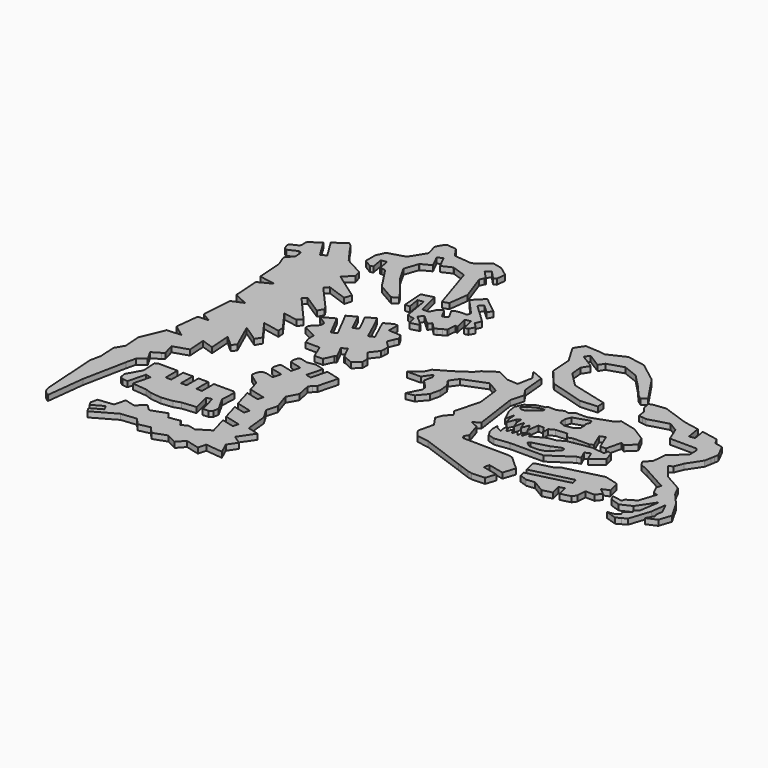
from build123d import *

# Parameters (mm, degrees)
F1_DEPTH = 3


# Not quite as in the source:
# - ends of sketch curves that miss each other by under 0.0002 mm in the source are joined


with BuildPart() as f1:
    # F0 (on Top) → F1 (new body)
    with BuildSketch(Plane.XY):
        Polygon((-104.437403, 46.564107), (-93.530615, 42.688137), (-92.321369, 46.634252), (-107.328489, 57.252365), (-102.324044, 61.359671), (-103.458085, 65.467584), (-113.663104, 70.984544), (-120.264377, 80.128426), (-120.756849, 80.974135), (-121.389462, 81.894522), (-122.514574, 83.041283), (-123.728328, 84.002663), (-130.063193, 79.125245), (-123.876212, 69.030337), (-126.463505, 67.191431), (-132.650487, 77.286339), (-137.732799, 73.674062), (-138.217282, 73.320664), (-138.526723, 72.785836), (-138.607686, 72.16178), (-138.468659, 70.035609), (-138.546917, 69.419841), (-138.847826, 68.889483), (-139.320957, 68.533506), (-142.435409, 67.101481), (-143.009225, 66.616569), (-143.281047, 65.887651), (-143.177988, 65.110044), (-142.393729, 63.132037), (-141.943435, 62.514076), (-141.266561, 62.221382), (-140.544494, 62.332335), (-136.10605, 64.373171), (-135.450674, 64.491083), (-134.818024, 64.272478), (-134.348725, 63.766009), (-134.147103, 63.084244), (-133.962555, 60.261903), (-134.064128, 59.580358), (-134.435555, 59.017782), (-136.792349, 56.777013), (-137.140032, 56.273256), (-137.268685, 55.661094), (-137.156299, 55.045254), (-135.022563, 49.646019), (-134.109418, 35.681092), (-125.140274, 34.118445), (-132.367969, 30.42543), (-131.412679, 15.815968), (-123.662433, 12.327511), (-129.911486, 9.725252), (-131.078484, -6.919091), (-125.924777, -10.012076), (-131.710451, -10.450802), (-133.125015, -23.174873), (-126.622962, -28.006874), (-134.303943, -28.589321), (-139.624962, -41.24429), (-138.992784, -50.912317), (-141.863543, -55.764821), (-141.271361, -64.821195), (-142.540436, -70.997637), (-140.515428, -101.966537), (-140.228003, -103.498246), (-139.58695, -104.900216), (-138.634739, -106.079438), (-137.434522, -106.957791), (-136.483255, -107.475311), (-134.012522, -86.428392), (-129.312015, -62.860274), (-128.020019, -57.445451), (-123.992793, -54.409686), (-127.09608, -48.956719), (-122.790594, -46.396882), (-121.548537, -45.29548), (-123.317555, -38.886306), (-115.18349, -36.282735), (-115.824054, -26.486441), (-109.192589, -28.71396), (-109.962426, -16.940676), (-104.125971, -22.186389), (-102.289088, -19.816338), (-108.825287, -5.250342), (-99.761113, -11.388933), (-97.77603, -7.98978), (-105.76927, 2.944957), (-96.452884, 1.068715), (-96.675299, 4.470164), (-104.586688, 15.321374), (-96.764237, 13.866803), (-94.584782, 16.079816), (-107.600103, 30.944294), (-105.732261, 32.840884), (-95.236183, 26.041835), (-93.454355, 29.231747), (-94.801805, 31.363182), (-106.496474, 44.528166), align=None)
    extrude(amount=F1_DEPTH)


with BuildPart() as f1b:
    # F0 (on Top) → F1, piece 2 (new body)
    with BuildSketch(Plane.XY):
        Polygon((-89.056032, 108.81387), (-89.684225, 108.642768), (-90.249705, 108.36248), (-90.766267, 107.966165), (-91.049446, 107.379957), (-92.740363, 104.245862), (-92.761765, 103.761682), (-92.617803, 103.298892), (-91.094478, 97.874397), (-96.342567, 89.382437), (-105.576906, 86.652048), (-107.737054, 81.985061), (-107.81263, 75.445893), (-103.524276, 72.84311), (-101.918124, 73.309127), (-103.032279, 79.807423), (-99.976868, 80.331274), (-98.921946, 74.178449), (-98.329958, 74.350211), (-95.800781, 73.792723), (-87.539001, 61.142449), (-83.059492, 58.556348), (-81.325187, 57.555105), (-78.121592, 55.705613), (-75.268916, 57.618377), (-77.57377, 61.251598), (-85.793508, 71.451888), (-90.559396, 79.785333), (-88.012588, 87.248984), (-87.488279, 87.697366), (-82.649191, 90.248926), (-85.944045, 96.896256), (-83.166522, 98.272979), (-79.871667, 91.625648), (-74.910829, 93.931576), (-74.236509, 94.077314), (-66.570524, 91.461465), (-58.372939, 65.993132), (-55.12332, 67.105068), (-53.747377, 77.891799), (-58.811761, 92.126912), (-57.723892, 94.477245), (-57.228728, 94.844348), (-57.275961, 94.894994), (-61.486422, 99.409668), (-59.219354, 101.523988), (-54.722596, 96.702332), (-53.37914, 97.698335), (-52.853684, 102.687158), (-54.477515, 103.893374), (-58.148833, 106.620508), (-63.146548, 107.678315), (-70.890179, 101.998314), (-80.826131, 102.964066), (-83.931775, 107.573558), (-84.212894, 107.968363), (-84.611172, 108.244523), (-88.418044, 108.684252), align=None)
    extrude(amount=F1_DEPTH)


with BuildPart() as f1c:
    # F0 (on Top) → F1, piece 3 (new body)
    with BuildSketch(Plane.XY):
        Polygon((-42.159712, 46.354486), (-40.319081, 47.369456), (-40.319496, 48.757673), (-40.035886, 52.328733), (-38.747849, 52.100388), (-38.657511, 52.126978), (-40.238607, 59.075176), (-37.215885, 59.763052), (-35.677786, 53.003806), (-33.794305, 53.558068), (-32.126363, 56.540318), (-34.89486, 59.272544), (-33.499978, 62.572179), (-38.761047, 67.63558), (-44.111875, 72.599139), (-42.003621, 74.871866), (-37.16445, 70.38293), (-35.646276, 72.995292), (-44.68013, 80.268067), (-50.226429, 74.695501), (-41.7868, 65.424247), (-42.380248, 63.371775), (-46.1018, 63.329178), (-48.125943, 62.914547), (-49.899462, 61.936585), (-47.046077, 56.762013), (-49.760707, 55.2651), (-52.614093, 60.439672), (-55.149767, 59.041439), (-56.932791, 55.347147), (-60.497214, 55.106867), (-63.550508, 67.348278), (-69.896804, 65.765349), (-69.05246, 53.912434), (-66.451193, 54.097766), (-67.567519, 60.669727), (-64.511289, 61.18887), (-62.162859, 47.517114), (-59.954925, 46.624454), (-59.968276, 46.648665), (-58.196369, 46.423521), (-57.009088, 42.030694), (-52.478271, 43.255272), (-52.267646, 43.553602), (-58.01691, 48.767286), (-55.934437, 51.063668), (-50.466297, 46.104917), (-49.090656, 48.053332), (-45.641155, 44.434734), (-44.429485, 45.102878), align=None)
    extrude(amount=F1_DEPTH)


with BuildPart() as f1d:
    # F0 (on Top) → F1, piece 4 (new body)
    with BuildSketch(Plane.XY):
        Polygon((-50.048866, 4.568951), (-53.825765, 9.290101), (-50.257894, 13.877362), (-50.048866, 16.092855), (-50.048866, 18.597474), (-53.825765, 22.374398), (-52.443705, 25.522427), (-51.397753, 27.904872), (-52.881541, 30.602621), (-59.49114, 31.007296), (-59.49114, 37.044992), (-61.447204, 37.044992), (-65.93857, 34.588814), (-60.398711, 22.505428), (-63.216676, 21.213468), (-68.665206, 33.097653), (-70.587792, 36.613251), (-75.208392, 34.086347), (-70.405513, 24.338759), (-73.186282, 22.968586), (-77.930728, 32.597564), (-82.763, 29.954908), (-81.268778, 27.222657), (-75.0956, 15.246371), (-77.851086, 13.826037), (-83.989445, 25.734784), (-90.380846, 22.239498), (-85.389947, 18.867223), (-85.389947, 16.574149), (-89.166846, 12.662325), (-89.166846, 10.639), (-81.747923, 7.131876), (-81.747923, 3.354952), (-80.53391, -0.017323), (-78.334601, -0.017323), (-76.277469, -0.017323), (-72.845212, -0.017323), (-69.74275, -7.436196), (-65.156501, -7.436196), (-62.863376, -2.310397), (-61.921049, -1.758048), (-65.426718, 5.301226), (-62.650225, 6.680051), (-59.240248, -0.186524), (-58.951577, -0.017323), (-53.825765, -2.310397), (-50.048866, 0.926927), align=None)
    extrude(amount=F1_DEPTH)


with BuildPart() as f1e:
    # F0 (on Top) → F1, piece 5 (new body)
    with BuildSketch(Plane.XY):
        Polygon((-75.430288, -23.271141), (-76.058576, -23.64166), (-76.264869, -23.909784), (-77.0207, -26.614304), (-77.013935, -27.343677), (-76.643403, -27.971962), (-76.008398, -28.330798), (-70.103598, -29.854618), (-71.240521, -34.260194), (-75.780919, -33.088478), (-76.878802, -33.0267), (-77.916726, -33.389771), (-78.736739, -34.122396), (-79.213925, -35.113052), (-79.74799, -37.182556), (-79.777736, -37.739591), (-79.588947, -38.264513), (-79.211233, -38.675058), (-73.457518, -42.851059), (-71.659574, -49.055771), (-62.769283, -51.35004), (-63.543907, -54.351707), (-70.656943, -52.516085), (-67.731057, -62.613493), (-59.56419, -64.721072), (-60.338813, -67.722734), (-66.728377, -66.073814), (-64.030647, -75.384005), (-55.411149, -77.608391), (-56.185772, -80.610053), (-63.027965, -78.844325), (-60.176841, -88.80404), (-67.161825, -93.110121), (-71.126836, -92.086892), (-74.615758, -93.770966), (-76.854063, -90.608898), (-82.986358, -91.610812), (-85.224663, -88.448743), (-93.74448, -91.418951), (-97.304474, -87.915814), (-99.0472, -89.68684), (-101.372527, -92.049925), (-107.149621, -90.559062), (-108.737669, -96.712747), (-116.966109, -97.643601), (-117.932495, -101.388347), (-116.718659, -103.538261), (-110.605866, -100.087016), (-109.081749, -102.786491), (-115.194543, -106.237737), (-113.740062, -108.81387), (-101.173814, -101.719032), (-92.657288, -100.862523), (-89.431274, -104.749365), (-82.965051, -103.363745), (-79.739037, -107.250587), (-72.491108, -104.657004), (-66.664429, -107.570357), (-63.047577, -103.569816), (-55.558085, -105.502588), (-54.421162, -101.097011), (-45.048666, -102.106025), (-47.848312, -95.838753), (-44.522848, -90.964192), (-49.278536, -87.719779), (-43.577011, -79.362376), (-49.68623, -77.785803), (-50.953558, -65.809785), (-54.385668, -59.990156), (-52.793977, -53.822356), (-55.707329, -45.082272), (-52.573661, -39.312395), (-54.115483, -31.663113), (-52.822456, -29.959439), (-51.223581, -28.618216), (-48.381276, -17.604286), (-51.163921, -16.886184), (-56.100521, -15.612223), (-58.356868, -24.355565), (-61.358527, -23.580943), (-59.102181, -14.837601), (-64.241319, -13.511372), (-66.810155, -13.998182), (-68.440858, -14.30721), (-72.142864, -13.351854), (-72.872212, -13.3586), (-73.500502, -13.729123), (-73.859368, -14.364144), (-74.462625, -16.701766), (-74.455861, -17.431139), (-74.085327, -18.05942), (-73.450323, -18.418259), (-67.545523, -19.942079), (-68.796138, -24.78821), (-74.700938, -23.264391), align=None)
    extrude(amount=F1_DEPTH)


with BuildPart() as f1f:
    # F0 (on Top) → F1, piece 6 (new body)
    with BuildSketch(Plane.XY):
        Polygon((-95.511904, -55.049836), (-95.512207, -63.250328), (-98.62354, -63.249836), (-98.622245, -55.049836), (-103.974963, -55.04899), (-103.976256, -63.233232), (-107.088527, -63.232729), (-107.087234, -55.048474), (-117.855523, -55.046772), (-119.091081, -55.832964), (-119.023882, -57.066132), (-118.908188, -59.189267), (-118.649276, -63.940604), (-122.921193, -71.627557), (-122.479558, -74.714973), (-120.877028, -75.844105), (-117.779126, -76.120585), (-115.302533, -66.371024), (-112.297975, -67.134254), (-114.651594, -76.39971), (-106.771164, -77.10302), (-103.128968, -78.336641), (-97.067074, -78.982632), (-91.00518, -78.336641), (-87.362985, -77.10302), (-79.482554, -76.39971), (-81.836173, -67.134254), (-78.831616, -66.371024), (-76.355023, -76.120585), (-73.257121, -75.844105), (-71.654591, -74.714973), (-71.212956, -71.627557), (-75.484872, -63.940604), (-75.043068, -55.832964), (-76.278625, -55.046772), (-87.046915, -55.048474), (-87.045621, -63.232729), (-90.157892, -63.233232), (-90.159186, -55.04899), align=None)
    extrude(amount=F1_DEPTH)


with BuildPart() as f1g:
    # F0 (on Top) → F1, piece 7 (new body)
    with BuildSketch(Plane.XY):
        Polygon((8.495949, -34.135969), (11.346512, -37.863053), (18.082474, -38.978129), (41.668499, -47.500932), (43.705116, -48.236862), (48.891428, -50.110934), (51.389669, -50.656791), (58.502406, -50.387424), (60.309291, -44.858784), (51.909904, -42.937152), (52.601264, -39.915215), (61.27627, -41.8999), (63.45597, -35.230399), (55.734619, -28.208075), (53.264095, -27.631666), (27.938087, -27.412399), (27.104545, -25.680222), (28.415999, -23.513753), (25.785276, -15.325359), (21.698488, -13.430989), (25.160498, -11.085757), (21.745718, 12.957322), (23.712684, 20.155122), (20.837889, 24.398867), (19.659859, 36.960822), (13.016846, 39.792383), (16.421207, 34.766897), (14.872141, 26.711679), (8.996459, 26.967452), (1.71219, 30.505123), (-4.876789, 26.041621), (-7.027485, 23.444219), (-14.398211, 18.451147), (-22.258862, 13.940791), (-23.620617, 10.900292), (-29.344982, 5.881985), (-21.93824, 6.011688), (-18.717606, 10.637306), (-17.582814, 8.962138), (-18.631145, 4.015904), (-14.106414, -0.739377), (-13.865017, -3.019809), (-17.478357, -10.192355), (-13.032845, -9.298961), (-8.7675, -4.291452), (-7.499394, 1.292387), (-7.94972, 6.52685), (-10.521909, 10.323891), (-7.448974, 14.686517), (5.159795, 19.643562), (11.435362, 15.911362), (12.948402, 3.57641), (9.345901, -10.105917), (11.388524, -13.121218), (8.256665, -16.248632), (6.818535, -20.090334), (10.510365, -25.540178), align=None)
    extrude(amount=F1_DEPTH)


with BuildPart() as f1h:
    # F0 (on Top) → F1, piece 8 (new body)
    with BuildSketch(Plane.XY):
        Polygon((46.31628, 74.243386), (36.435113, 76.041081), (32.979415, 74.41313), (31.25546, 73.60099), (26.861843, 71.531194), (23.451776, 72.049742), (15.694626, 72.513066), (12.388123, 67.488849), (18.404778, 57.332014), (19.164542, 45.733344), (26.766633, 36.64906), (45.655597, 31.14136), (54.887635, 31.772631), (54.588393, 35.997475), (34.948236, 41.071774), (27.038098, 48.984554), (26.513995, 55.362823), (28.986028, 59.29483), (21.286694, 64.135364), (22.936641, 66.759792), (30.635984, 61.919269), (32.539838, 64.947517), (41.341244, 67.724972), (49.551788, 64.506242), (56.573036, 57.271918), (62.09137, 50.832995), (64.609843, 48.910836), (67.255221, 50.994557), (57.279075, 65.876312), align=None)
    extrude(amount=F1_DEPTH)


with BuildPart() as f1i:
    # F0 (on Top) → F1, piece 9 (new body)
    with BuildSketch(Plane.XY):
        Polygon((41.50084, -4.359526), (43.008741, -0.46998), (43.68228, -1.009414), (45.119556, -4.359526), (46.019556, 1.951114), (49.058002, 1.951114), (51.395266, -1.554777), (51.395266, 1.951114), (54.199987, 3.431378), (60.354797, 3.976741), (62.458336, 1.016213), (65.496782, 1.951114), (68.825445, 1.951114), (71.163095, 1.951114), (74.300488, 1.951114), (75.867294, 2.789517), (72.620786, 10.525798), (75.462236, 11.718197), (78.960044, 3.383076), (82.013472, 3.431378), (84.039104, 11.767645), (86.064737, 10.59903), (90.661362, 15.039822), (87.934551, 20.415561), (80.377386, 25.167957), (71.339949, 27.349454), (69.080591, 25.167957), (67.033284, 24.443741), (61.209136, 22.383503), (57.627983, 21.116703), (51.473178, 21.116703), (48.980089, 19.013187), (46.487006, 19.714374), (43.02313, 18.078286), (38.462388, 18.078286), (37.917025, 17.221274), (36.313726, 16.840829), (35.521631, 16.652874), (33.320403, 16.130548), (28.9575, 13.17002), (27.087686, 9.118721), (27.358255, 7.224767), (27.710961, 4.755863), (30.784317, -1.851861), (32.072677, 3.04184), (32.38549, -1.009414), (33.398304, -4.359526), (35.190217, 0.427862), (36.904212, 1.951114), (36.904212, -1.554777), (38.384481, -5.13858), (39.708932, 0.315026), align=None)
        Polygon((29.249174, 10.309388), (31.293509, 12.503303), (35.830915, 14.796977), (36.632082, 14.930491), (38.822621, 15.295543), (38.822621, 14.198562), (38.024831, 13.301053), (32.340599, 9.15972), (30.482975, 9.15972), align=None, mode=Mode.SUBTRACT)
        Polygon((51.33145, 13.950375), (52.488246, 16.782518), (61.209136, 19.603975), (61.981914, 17.739882), (61.024573, 15.545967), (61.622908, 14.548699), (61.622908, 11.51713), (58.910436, 9.56259), (54.522605, 8.764748), (51.810126, 10.001345), (51.33145, 11.51713), align=None, mode=Mode.SUBTRACT)
    extrude(amount=F1_DEPTH)


with BuildPart() as f1j:
    # F0 (on Top) → F1, piece 10 (new body)
    with BuildSketch(Plane.XY):
        Polygon((51.059302, -18.357568), (59.964344, -18.357568), (65.195759, -18.357568), (76.975585, -10.442045), (79.165727, -9.940283), (77.102139, -5.395955), (79.907909, -4.121837), (82.061186, -8.863711), (88.194471, -4.006741), (86.885603, 0.963845), (84.527343, 1.894318), (84.205535, -0.594354), (76.975585, 0.340593), (71.437985, -0.620036), (69.089892, -1.027368), (64.759469, -1.778583), (60.583551, -4.006741), (56.24399, -4.610201), (49.20885, -8.447556), (47.806486, -5.876589), (46.559942, -9.908348), (44.941527, -7.434742), (44.641527, -10.784832), (42.586595, -8.126655), (41.494687, -10.784832), (39.937687, -7.434742), (38.613236, -10.784832), (36.576486, -7.434742), (35.964334, -9.226655), (36.576486, -12.178874), (34.873603, -11.208348), (33.704976, -10.784832), (32.536338, -9.226655), (32.536338, -13.281105), (33.083459, -15.280503), (34.873603, -18.264087), (38.613236, -19.354813), (46.559942, -18.357568), align=None)
        Polygon((68.497801, -9.978361), (63.075206, -14.71497), (59.964344, -15.540834), (59.064344, -15.540834), (54.964344, -15.540834), (52.32196, -13.564017), (53.220513, -12.362933), (62.00253, -9.978361), (66.597801, -8.007705), (68.497801, -8.007705), align=None, mode=Mode.SUBTRACT)
    extrude(amount=F1_DEPTH)


with BuildPart() as f1k:
    # F0 (on Top) → F1, piece 11 (new body)
    with BuildSketch(Plane.XY):
        Polygon((108.160437, -0.992934), (122.396546, -8.860139), (121.591766, -11.434516), (123.833573, -15.823861), (126.105971, -16.559774), (123.119026, -25.783044), (118.211248, -28.624362), (117.648493, -30.362074), (112.121376, -29.369647), (113.388281, -32.02482), (118.842007, -33.791003), (124.825523, -31.002687), (131.213632, -21.492594), (129.530734, -32.526463), (127.092516, -34.218031), (128.053614, -35.603361), (124.537503, -38.042667), (125.222426, -39.992608), (123.303718, -41.852425), (119.235861, -42.425474), (125.216993, -44.362456), (127.712364, -43.002451), (130.248424, -41.62027), (133.988597, -30.07113), (135.054188, -21.672983), (137.877109, -27.549559), (137.410574, -31.179332), (138.026664, -32.56037), (135.609749, -36.740032), (141.133908, -34.275556), (143.281046, -27.645492), (137.867299, -18.094237), (131.836242, -11.178709), (129.197103, -6.011493), (119.253669, -0.392921), (113.118121, 7.360964), (115.165354, 8.536061), (117.14957, 13.433531), (122.195723, 21.125375), (122.841526, 24.646715), (123.241677, 26.828595), (123.609476, 28.834075), (120.091161, 35.721363), (115.859521, 36.497995), (113.938097, 39.824483), (104.886855, 41.541735), (105.981261, 34.970489), (102.923359, 34.461212), (101.641593, 42.157445), (93.228042, 43.753711), (79.161368, 48.675499), (72.660318, 47.934626), (70.429792, 47.221302), (71.029939, 43.617782), (73.408754, 40.452914), (74.1243, 36.156485), (76.343651, 35.85302), (78.351349, 35.578495), (89.508504, 38.718642), (94.589905, 35.576548), (97.730447, 27.838042), (112.421375, 27.720771), (113.631996, 26.448645), (113.728721, 21.481982), (105.812315, 14.669926), (105.234177, 7.209804), (101.982299, 3.561181), (103.311269, 1.245875), align=None)
    extrude(amount=F1_DEPTH)


with BuildPart() as f1l:
    # F0 (on Top) → F1, piece 12 (new body)
    with BuildSketch(Plane.XY):
        Polygon((88.489248, -37.262785), (91.496958, -36.512222), (92.839596, -41.892536), (98.242354, -40.544298), (99.760677, -38.448952), (100.067968, -33.14468), (105.047758, -33.273421), (107.454028, -30.365134), (103.886869, -27.413708), (107.867221, -25.839719), (106.282746, -19.490298), (105.101156, -18.958746), (98.620181, -17.315706), (78.201039, -22.411229), (75.966096, -24.278488), (75.474258, -24.401224), (74.98242, -24.52396), (72.320098, -25.188334), (66.501346, -26.640382), (66.213603, -27.246657), (67.692439, -33.172752), (90.273205, -27.537805), (91.02378, -30.545562), (68.484148, -36.170246), (69.243239, -39.212131), (73.405322, -40.627724), (77.9721, -40.134664), (84.641606, -44.140209), (89.879314, -42.833158), align=None)
    extrude(amount=F1_DEPTH)


solid = Compound([f1.part, f1b.part, f1c.part, f1d.part, f1e.part, f1f.part, f1g.part, f1h.part, f1i.part, f1j.part, f1k.part, f1l.part])
